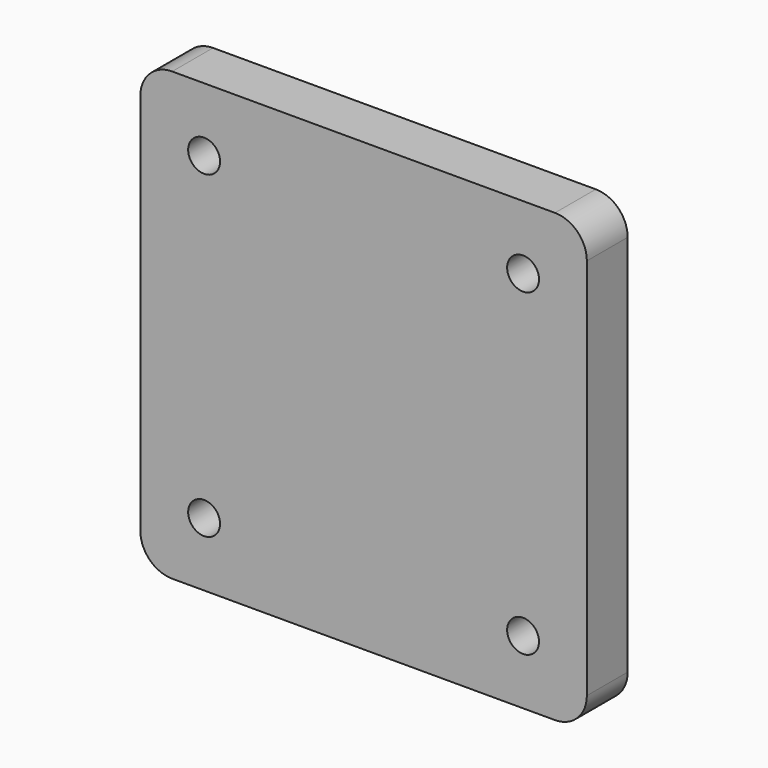
from build123d import *

# Parameters (mm, degrees)
F0_R     = 2.5
F1_DEPTH = 4


# Not quite as in the source:
# - a pattern or mirror of a feature is missing from the dataset's text; its kind, count and spacing are read off the source's solid


with BuildPart() as f1:
    # F0 (on Front) → F1 (new body)
    with BuildSketch(Plane.XZ):
        with BuildLine():
            Line((30, 35), (-30, 35))
            ThreePointArc((-30, 35), (-33.5355339059, 33.5355339059), (-35, 30))
            Line((-35, 30), (-35, -30))
            ThreePointArc((-35, -30), (-33.5355339059, -33.5355339059), (-30, -35))
            Line((-30, -35), (30, -35))
            ThreePointArc((30, -35), (33.5355339059, -33.5355339059), (35, -30))
            Line((35, -30), (35, 30))
            ThreePointArc((35, 30), (33.5355339059, 33.5355339059), (30, 35))
        make_face()
        with Locations((-25, -25)):
            Circle(F0_R, mode=Mode.SUBTRACT)
        with Locations((25, -25)):
            Circle(F0_R, mode=Mode.SUBTRACT)
        with Locations((-25, 25)):
            Circle(F0_R, mode=Mode.SUBTRACT)
        with Locations((25, 25)):
            Circle(F0_R, mode=Mode.SUBTRACT)
    extrude(amount=F1_DEPTH)

    # F1_copies: F1 across plane


with BuildPart() as f1_1:
    add(f1.part)
    add(f1.part.mirror(Plane(origin=(0, -4, 0), x_dir=(0, 0, -1), z_dir=(0, -1, 0))))


solid = f1_1.part
